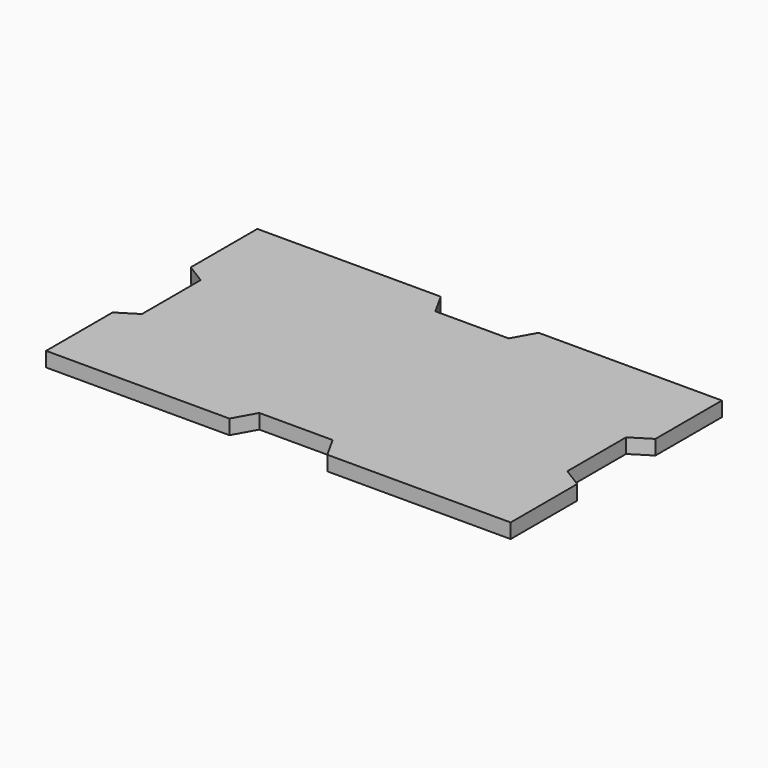
from build123d import *

# Parameters (mm, degrees)
F0_W     = 37.5
F0_H     = 17
F1_DEPTH = 3


# Not quite as in the source:
# - a feature names something its author has since deleted; it is built from what else it names


with BuildPart() as f1:
    # F0 (on Top) → F1 (new body)
    with BuildSketch(Plane.XY):
        with Locations((18.75, 45.5)):
            Rectangle(F0_W, F0_H)
        Polygon((95, 37), (37.5, 37), (37.5, 0), (40, 4.5), (47.5, 4.5), (55, 4.5), (57.5, 0), (95, 0), (95, 17), (91, 19.5), (91, 27), (91, 34.5), align=None)
        Polygon((40, 49.5), (37.5, 54), (37.5, 37), (95, 37), (95, 54), (57.5, 54), (55, 49.5), (47.5, 49.5), align=None)
        Polygon((37.5, 37), (0, 37), (4, 34.5), (4, 27), (4, 19.5), (0, 17), (0, 0), (37.5, 0), align=None)
    extrude(amount=F1_DEPTH)


solid = f1.part
